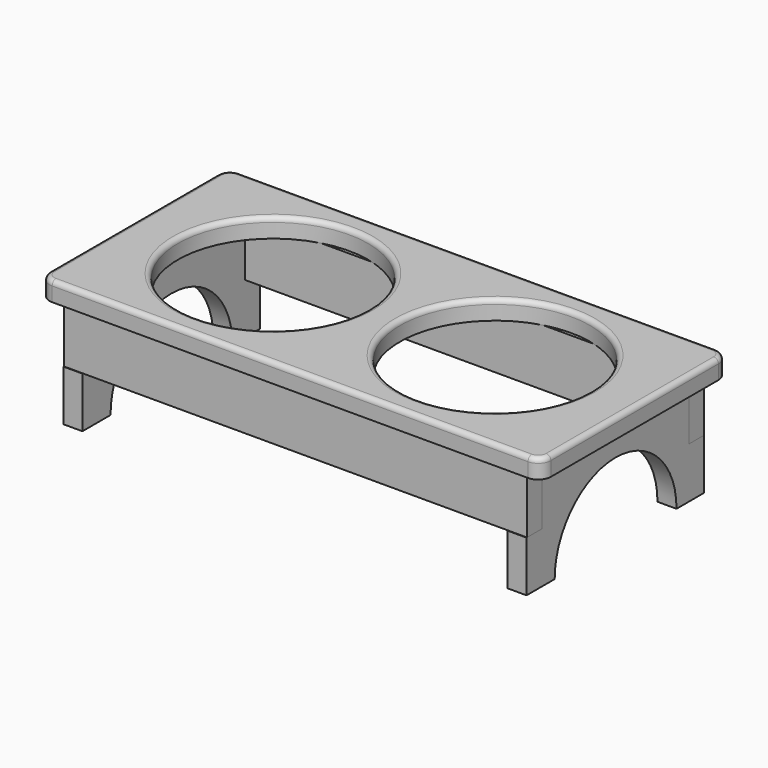
from build123d import *

# Parameters (mm, degrees)
F0_R     = 95.25
F1_DEPTH = 19.05
F2_R     = 4.7625
F4_DEPTH = 19.05
F5_W     = 463.55
F5_H     = 57.15
F6_DEPTH = 19.05


with BuildPart() as f1:
    # F0 (on Top) → F1 (new body)
    with BuildSketch(Plane.XY):
        with BuildLine():
            Line((0, -117.475), (0, 117.475))
            Line((0, 117.475), (-238.125, 117.475))
            ThreePointArc((-238.125, 117.475), (-247.1052561211, 113.7552561211), (-250.825, 104.775))
            Line((-250.825, 104.775), (-250.825, -104.775))
            ThreePointArc((-250.825, -104.775), (-247.1052561211, -113.7552561211), (-238.125, -117.475))
            Line((-238.125, -117.475), (0, -117.475))
        make_face()
        with Locations((-111.125, 0)):
            Circle(F0_R, mode=Mode.SUBTRACT)
        with BuildLine():
            Line((238.125, 117.475), (0, 117.475))
            Line((0, 117.475), (0, -117.475))
            Line((0, -117.475), (238.125, -117.475))
            ThreePointArc((238.125, -117.475), (247.1052561211, -113.7552561211), (250.825, -104.775))
            Line((250.825, -104.775), (250.825, 104.775))
            ThreePointArc((250.825, 104.775), (247.1052561211, 113.7552561211), (238.125, 117.475))
        make_face()
        with Locations((111.125, 0)):
            Circle(F0_R, mode=Mode.SUBTRACT)
    extrude(amount=F1_DEPTH)

    # F2
    f2_edges = [f1.edges().sort_by_distance(p)[0] for p in [
        (0, -117.475, 19.05),
        (-206.375, 0, 19.05),
        (15.875, 0, 19.05),
        (247.105256, -113.755256, 19.05),
        (250.825, 0, 19.05),
        (247.105256, 113.755256, 19.05),
        (0, 117.475, 19.05),
        (-247.105256, 113.755256, 19.05),
        (-250.825, 0, 19.05),
        (-247.105256, -113.755256, 19.05),
    ]]
    fillet(f2_edges, radius=F2_R)


with BuildPart() as f4:
    # F3 (on Right) → F4 (new body)
    with BuildSketch(Plane.YZ):
        with BuildLine():
            Line((92.329, 0), (-92.329, 0))
            Line((-92.329, 0), (-92.329, -57.15))
            Line((-92.329, -57.15), (-111.379, -57.15))
            Line((-111.379, -57.15), (-111.379, -107.95))
            Line((-111.379, -107.95), (-76.2, -107.95))
            ThreePointArc((-76.2, -107.95), (0, -31.75), (76.2, -107.95))
            Line((76.2, -107.95), (110.871, -107.95))
            Line((110.871, -107.95), (110.871, -57.15))
            Line((110.871, -57.15), (92.329, -57.15))
            Line((92.329, -57.15), (92.329, 0))
        make_face()
    extrude(amount=F4_DEPTH)


with BuildPart() as f6:
    # F5 (on Front) → F6 (new body)
    with BuildSketch(Plane.XZ):
        with Locations((0, -28.575)):
            Rectangle(F5_W, F5_H)
    extrude(amount=F6_DEPTH)


with BuildPart() as f4_1:
    # F7: moved
    add(f4.part.moved(Location((-231.775, 0, 0))))


with BuildPart() as f8_1:
    # F8: instance of F4
    add(f4_1.part.mirror(Plane.YZ))


with BuildPart() as f6_1:
    # F9: moved
    add(f6.part.moved(Location((0, 110.871, 0))))


with BuildPart() as f10_1:
    # F10: instance of F6
    add(f6_1.part.mirror(Plane.XZ))


solid = Compound([f1.part, f4_1.part, f8_1.part, f6_1.part, f10_1.part])
